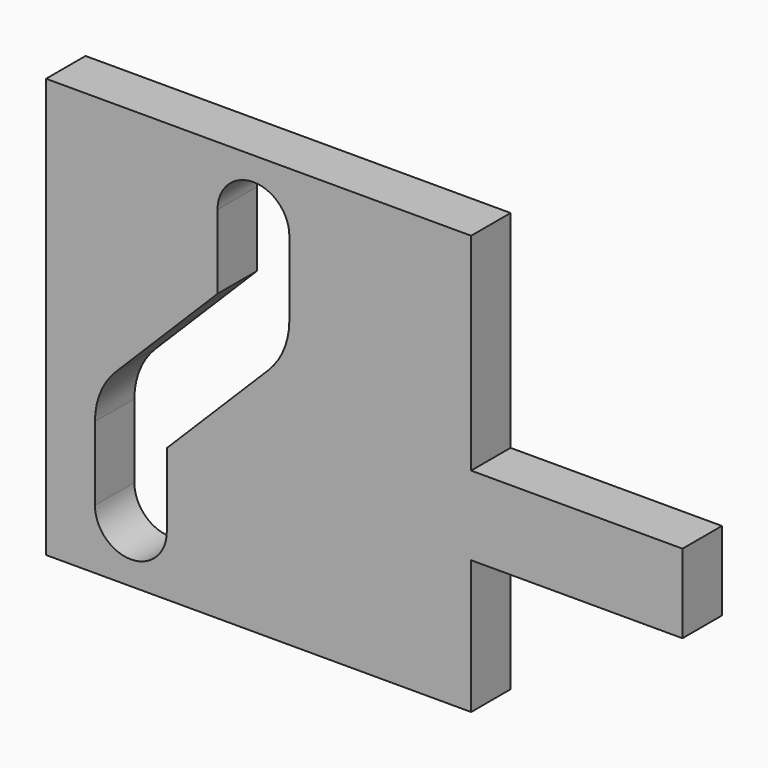
from build123d import *

# Parameters (mm, degrees)
F1_DEPTH = 8.89


# Not quite as in the source:
# - ends of sketch curves that miss each other by under 0.0002 mm in the source are joined


with BuildPart() as f1:
    # F0 (on Front) → F1 (new body)
    with BuildSketch(Plane.XZ):
        Polygon((49.2809079587, 38.859821856), (0, 38.859821856), (-27.3745507002, 38.859821856), (-27.3745507002, 1.9207646612), (-27.3745507002, -36.7616191506), (49.2809079587, -36.7616191506), (49.2809079587, -12.6536535591), (87.395709982, -12.6536535591), (87.395709982, -5.5416535591), (87.395709982, 1.5703464409), (49.2809079587, 1.5703464409), align=None)
        with BuildLine():
            Line((-5.6126600757, 5.6126600757), (0, 11.2253201513))
            Line((0, 11.2253201513), (3.5468912197, 14.7722113711))
            Line((3.5468912197, 14.7722113711), (3.5468912197, 28.1402313711))
            ThreePointArc((3.5468912197, 28.1402313711), (10.0238912197, 34.6172313711), (16.5008912197, 28.1402313711))
            Line((16.5008912197, 28.1402313711), (16.5008912197, 14.7722113711))
            ThreePointArc((16.5008912197, 14.7722113711), (15.5148266839, 9.8149301882), (12.7067524632, 5.6123501276))
            Line((12.7067524632, 5.6123501276), (3.5517127264, -3.5426896092))
            Line((3.5517127264, -3.5426896092), (-5.6081485171, -12.7025508527))
            Line((-5.6081485171, -12.7025508527), (-5.6081485171, -26.002401486))
            ThreePointArc((-5.6081485171, -26.002401486), (-12.085148378, -32.479401347), (-18.562148239, -26.002401486))
            Line((-18.562148239, -26.002401486), (-18.562148239, -12.7025505746))
            ThreePointArc((-18.562148239, -12.7025505746), (-17.5773042343, -7.7482170412), (-14.7725202074, -3.5472022785))
            Line((-14.7725202074, -3.5472022785), (-14.7680094825, -3.5426893311))
            Line((-14.7680094825, -3.5426893311), (-5.6129700238, 5.6123501276))
            Line((-5.6129700238, 5.6123501276), (-5.6126600757, 5.6126600757))
        make_face(mode=Mode.SUBTRACT)
    extrude(amount=F1_DEPTH)


solid = f1.part
